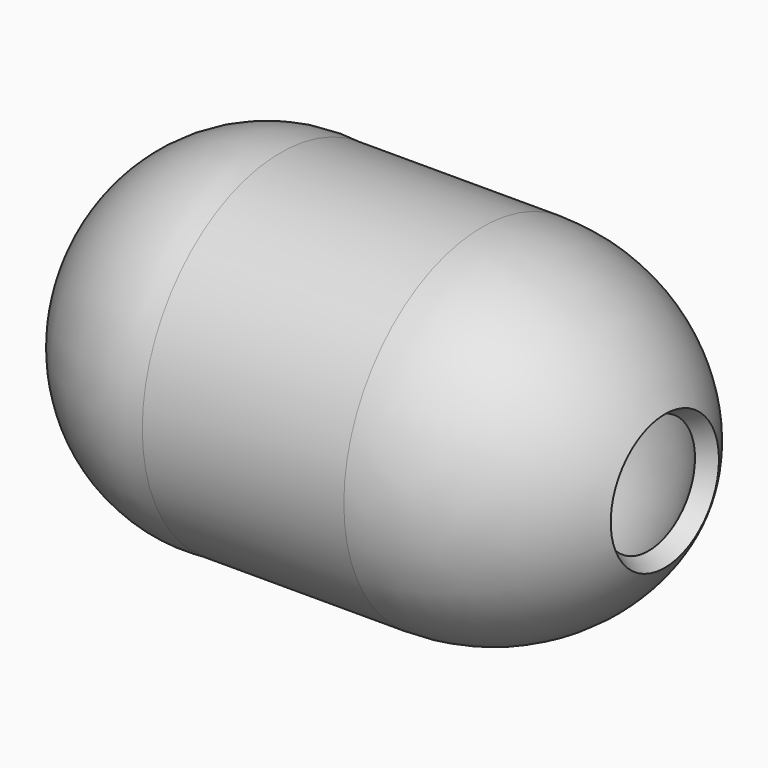
from build123d import *


# Not quite as in the source:
# - ends of sketch curves that miss each other by under 0.0002 mm in the source are joined


with BuildPart() as f1:
    # F0 (on Top) → F1 (revolve)
    with BuildSketch(Plane.XY):
        with BuildLine():
            ThreePointArc((-89.0986546874, 19.8162570596), (-69.1779558985, 44.6400212025), (-38.1425693631, 51.7010614276))
            Line((-38.1425693631, 51.7010614276), (29.7988802195, 51.7010614276))
            ThreePointArc((29.7988802195, 51.7010614276), (61.97374073, 43.0773793158), (85.5227932334, 19.518269226))
            Line((85.5227932334, 19.518269226), (91.022959273, 22.6917042953))
            ThreePointArc((91.022959273, 22.6917042953), (65.1495240793, 48.5761897981), (29.7988802195, 58.0510627349))
            Line((29.7988802195, 58.0510627349), (-37.7985022652, 58.0510608852))
            ThreePointArc((-37.7985022652, 58.0510608852), (-72.7012317245, 49.9257206617), (-95.0833715048, 21.9389113347))
            Line((-95.0833715048, 21.9389113347), (-89.0986546874, 19.8162570596))
        make_face()
    revolve(axis=Axis((-4.6188272536, 0, 0), (1, 0, 0)))


solid = f1.part
